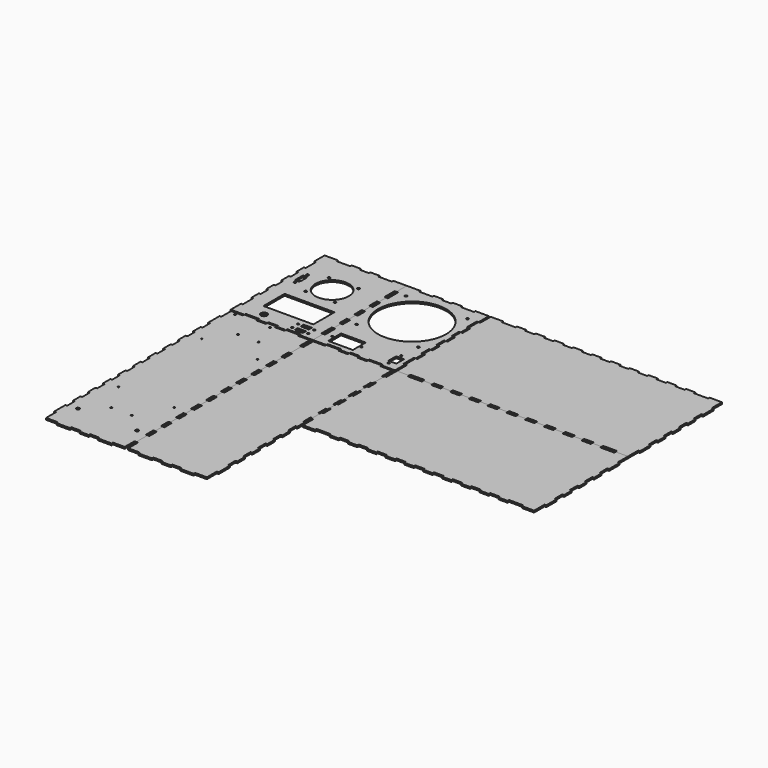
from build123d import *

# Parameters (mm, degrees)
F0_R     = 5.5001224188
F0_R_2   = 1.7501355185
F0_W     = 14
F0_H     = 6.5
F0_W_2   = 85
F0_H_2   = 45
F0_R_3   = 2.2023972195
F0_R_4   = 1.9999459509
F0_R_5   = 28.5
F1_DEPTH = 3
F0_R_6   = 2.75
F0_R_7   = 1.5
F0_R_8   = 1.25
F0_R_9   = 1.5001561361
F2_DEPTH = 3
F0_R_10  = 1.4999539677
F0_W_3   = 42
F0_H_3   = 27.5
F0_R_11  = 1.75
F0_W_4   = 13.5
F0_H_4   = 16.5
F0_R_12  = 1.9998336797
F0_R_13  = 58
F3_DEPTH = 3
F4_DEPTH = 3
F5_DEPTH = 3
F6_DEPTH = 3


# Not quite as in the source:
# - ends of sketch curves that miss each other by under 0.0002 mm in the source are joined


with BuildPart() as f1:
    # F0 (on Top) → F1 (new body)
    with BuildSketch(Plane.XY):
        Polygon((-317.001144, 300.00067), (-340.00059, 300.00067), (-340.00059, 278.00173), (-337.000596, 278.00173), (-337.000596, 256.00279), (-340.00059, 256.00279), (-340.00059, 240.00079), (-337.000596, 240.00079), (-337.000596, 223.99879), (-340.00059, 223.99879), (-340.00059, 207.99933), (-337.000596, 207.99933), (-337.000596, 191.99733), (-340.00059, 191.99733), (-340.00059, 175.99787), (-337.000596, 175.99787), (-337.000596, 159.99587), (-340.00059, 159.99587), (-340.00059, 144.00149), (-337.000596, 144.00149), (-337.000596, 122.00001), (-340.00059, 122.00001), (-340.00059, 100.00107), (-317.001144, 100.00107), (-317.001144, 102.99827), (-294.000174, 102.99827), (-294.000174, 100.00107), (-278.001222, 100.00107), (-278.001222, 102.99827), (-262.000746, 102.99827), (-262.000746, 100.00107), (-246.000524, 100.00107), (-246.000524, 102.99827), (-223.001078, 102.99827), (-223.001078, 100.00107), (-200.000108, 100.00107), (-200.000108, 122.00001), (-203.000102, 122.00001), (-203.000102, 144.00149), (-200.000108, 144.00149), (-200.000108, 159.99587), (-203.000102, 159.99587), (-203.000102, 175.99787), (-200.000108, 175.99787), (-200.000108, 191.99733), (-203.000102, 191.99733), (-203.000102, 207.99933), (-200.000108, 207.99933), (-200.000108, 223.99879), (-203.000102, 223.99879), (-203.000102, 240.00079), (-200.000108, 240.00079), (-200.000108, 256.00279), (-203.000102, 256.00279), (-203.000102, 278.00173), (-200.000108, 278.00173), (-200.000108, 300.00067), (-223.001078, 300.00067), (-223.001078, 297.00093), (-246.000524, 297.00093), (-246.000524, 300.00067), (-262.000746, 300.00067), (-262.000746, 297.00093), (-278.001222, 297.00093), (-278.001222, 300.00067), (-294.000174, 300.00067), (-294.000174, 297.00093), (-317.001144, 297.00093), align=None)
        with Locations((-296.856862573, 116.9972511531)):
            Circle(F0_R, mode=Mode.SUBTRACT)
        with Locations((-243.809402042, 110.6649048161)):
            Circle(F0_R_2, mode=Mode.SUBTRACT)
        with Locations((-230.059402042, 110.6915399432)):
            Rectangle(F0_W, F0_H, mode=Mode.SUBTRACT)
        with Locations((-216.309402042, 110.6649048161)):
            Circle(F0_R_2, mode=Mode.SUBTRACT)
        with Locations((-243.8093970094, 123.4562702011)):
            Circle(F0_R_2, mode=Mode.SUBTRACT)
        with Locations((-230.0593970094, 123.4829053283)):
            Rectangle(F0_W, F0_H, mode=Mode.SUBTRACT)
        with Locations((-216.3093970094, 123.4562702011)):
            Circle(F0_R_2, mode=Mode.SUBTRACT)
        with Locations((-270.001013279, 157.8700011969)):
            Rectangle(F0_W_2, F0_H_2, mode=Mode.SUBTRACT)
        with Locations((-322.4638801523, 215.0738120902)):
            Circle(F0_R_3, mode=Mode.SUBTRACT)
        with Locations((-295.0011516983, 203.4637744319)):
            Circle(F0_R_4, mode=Mode.SUBTRACT)
        with Locations((-245.0010429199, 203.4637744319)):
            Circle(F0_R_4, mode=Mode.SUBTRACT)
        Polygon((-318.3998801523, 222.5198170102), (-320.1778801523, 219.7258170102), (-326.5278801523, 219.7258170102), (-326.5278801523, 237.2258175702), (-320.1778801523, 237.2258175702), (-318.3998801523, 234.4318175702), align=None, mode=Mode.SUBTRACT)
        with Locations((-322.4638801523, 241.8778224902)):
            Circle(F0_R_3, mode=Mode.SUBTRACT)
        with Locations((-270.0010973091, 228.4637673539)):
            Circle(F0_R_5, mode=Mode.SUBTRACT)
        with Locations((-295.0011516983, 253.4637602758)):
            Circle(F0_R_4, mode=Mode.SUBTRACT)
        with Locations((-245.0010429199, 253.4637602758)):
            Circle(F0_R_4, mode=Mode.SUBTRACT)
    extrude(amount=F1_DEPTH)


with BuildPart() as f2:
    # F0 (on Top) → F2 (new body)
    with BuildSketch(Plane.XY):
        Polygon((-294.000174, 100.00107), (-317.001144, 100.00107), (-317.001144, 96.99879), (-337.000596, 96.99879), (-337.000596, 76.00061), (-340.00059, 76.00061), (-340.00059, 52.00015), (-337.000596, 52.00015), (-337.000596, 35.99815), (-340.00059, 35.99815), (-340.00059, 20.00123), (-337.000596, 20.00123), (-337.000596, 3.99923), (-340.00059, 3.99923), (-340.00059, -12.00023), (-337.000596, -12.00023), (-337.000596, -28.00223), (-340.00059, -28.00223), (-340.00059, -43.99915), (-337.000596, -43.99915), (-337.000596, -60.001404), (-340.00059, -60.001404), (-340.00059, -76.00061), (-337.000596, -76.00061), (-337.000596, -92.001086), (-340.00059, -92.001086), (-340.00059, -108.000038), (-337.000596, -108.000038), (-337.000596, -124.00153), (-340.00059, -124.00153), (-340.00059, -139.999466), (-337.000596, -139.999466), (-337.000596, -156.000958), (-340.00059, -156.000958), (-340.00059, -172.000164), (-337.000596, -172.000164), (-337.000596, -188.00191), (-340.00059, -188.00191), (-340.00059, -203.999592), (-337.000596, -203.999592), (-337.000596, -220.001338), (-340.00059, -220.001338), (-340.00059, -236.000544), (-337.000596, -236.000544), (-337.000596, -252.000766), (-340.00059, -252.000766), (-340.00059, -276.000718), (-337.0006056227, -276.000718), (-337.000596, -297.000676), (-317.001144, -297.000676), (-317.001144, -300.00067), (-294.000174, -300.00067), (-294.000174, -297.000676), (-278.001222, -297.000676), (-278.001222, -300.00067), (-262.000746, -300.00067), (-262.000746, -297.000676), (-246.000524, -297.000676), (-246.000524, -300.00067), (-223.001078, -300.00067), (-223.001078, -297.000676), (-203.000102, -297.000676), (-203.000102, -276.000718), (-200.000108, -276.000718), (-200.000108, -252.000766), (-203.000102, -252.000766), (-203.000102, -236.000544), (-200.000108, -236.000544), (-200.000108, -220.001338), (-203.000102, -220.001338), (-203.000102, -203.999592), (-200.000108, -203.999592), (-200.000108, -188.00191), (-203.000102, -188.00191), (-203.000102, -172.000164), (-200.000108, -172.000164), (-200.000108, -156.000958), (-203.000102, -156.000958), (-203.000102, -139.999466), (-200.000108, -139.999466), (-200.000108, -124.00153), (-203.000102, -124.00153), (-203.000102, -108.000038), (-200.000108, -108.000038), (-200.000108, -92.001086), (-203.000102, -92.001086), (-203.000102, -76.00061), (-200.000108, -76.00061), (-200.000108, -60.001404), (-203.000102, -60.001404), (-203.000102, -43.99915), (-200.000108, -43.99915), (-200.000108, -28.00223), (-203.000102, -28.00223), (-203.000102, -12.00023), (-200.000108, -12.00023), (-200.000108, 3.99923), (-203.000102, 3.99923), (-203.000102, 20.00123), (-200.000108, 20.00123), (-200.000108, 35.99815), (-203.000102, 35.99815), (-203.000102, 52.00015), (-200.000108, 52.00015), (-200.000108, 76.00061), (-203.000102, 76.00061), (-203.000102, 96.99879), (-223.001078, 96.99879), (-223.001078, 100.00107), (-246.000524, 100.00107), (-246.000524, 96.99879), (-262.000746, 96.99879), (-262.000746, 100.00107), (-278.001222, 100.00107), (-278.001222, 96.99879), (-294.000174, 96.99879), align=None)
        with Locations((-320.4981392353, -249.8400263762)):
            Circle(F0_R_6, mode=Mode.SUBTRACT)
        with Locations((-219.4981392353, -249.8400263762)):
            Circle(F0_R_6, mode=Mode.SUBTRACT)
        with Locations((-287.4827867562, -219.9880003408)):
            Circle(F0_R_7, mode=Mode.SUBTRACT)
        with Locations((-317.5006971111, -167.2832300663)):
            Circle(F0_R_8, mode=Mode.SUBTRACT)
        with Locations((-252.4827370386, -219.9884861494)):
            Circle(F0_R_7, mode=Mode.SUBTRACT)
        with Locations((-222.5006971111, -167.2832300663)):
            Circle(F0_R_8, mode=Mode.SUBTRACT)
        with Locations((-317.5006971111, 10.2167699337)):
            Circle(F0_R_8, mode=Mode.SUBTRACT)
        with Locations((-287.483402451, 50.0039782226)):
            Circle(F0_R_7, mode=Mode.SUBTRACT)
        with Locations((-222.5006971111, 10.2167699337)):
            Circle(F0_R_8, mode=Mode.SUBTRACT)
        with Locations((-252.4833581656, 50.0046229419)):
            Circle(F0_R_7, mode=Mode.SUBTRACT)
        with Locations((-326.6070187092, 92.3456028104)):
            Circle(F0_R_9, mode=Mode.SUBTRACT)
        with Locations((-267.1067064369, 92.3456028104)):
            Circle(F0_R_9, mode=Mode.SUBTRACT)
    extrude(amount=F2_DEPTH)


with BuildPart() as f3:
    # F0 (on Top) → F3 (new body)
    with BuildSketch(Plane.XY):
        Polygon((-177.000662, 300.00067), (-200.000108, 300.00067), (-200.000108, 278.00173), (-197.000368, 278.00173), (-197.000368, 256.00279), (-200.000108, 256.00279), (-200.000108, 240.00079), (-197.000368, 240.00079), (-197.000368, 223.99879), (-200.000108, 223.99879), (-200.000108, 207.99933), (-197.000368, 207.99933), (-197.000368, 191.99733), (-200.000108, 191.99733), (-200.000108, 175.99787), (-197.000368, 175.99787), (-197.000368, 159.99587), (-200.000108, 159.99587), (-200.000108, 144.00149), (-197.000368, 144.00149), (-197.000368, 122.00001), (-200.000108, 122.00001), (-200.000108, 100.00107), (-177.000662, 100.00107), (-177.000662, 102.99827), (-154.001216, 102.99827), (-154.001216, 100.00107), (-138.00074, 100.00107), (-138.00074, 102.99827), (-122.000518, 102.99827), (-122.000518, 100.00107), (-105.999788, 100.00107), (-105.999788, 102.99827), (-83.00085, 102.99827), (-83.00085, 100.00107), (-60.00115, 100.00107), (-60.00115, 122.00001), (-63.00089, 122.00001), (-63.00089, 144.00149), (-60.00115, 144.00149), (-60.00115, 159.99587), (-63.00089, 159.99587), (-63.00089, 175.99787), (-60.00115, 175.99787), (-60.00115, 191.99733), (-63.00089, 191.99733), (-63.00089, 207.99933), (-60.00115, 207.99933), (-60.00115, 223.99879), (-63.00089, 223.99879), (-63.00089, 240.00079), (-60.00115, 240.00079), (-60.00115, 256.00279), (-63.00089, 256.00279), (-63.00089, 278.00173), (-60.00115, 278.00173), (-60.00115, 300.00067), (-83.00085, 300.00067), (-83.00085, 297.00093), (-105.999788, 297.00093), (-105.999788, 300.00067), (-122.000518, 300.00067), (-122.000518, 297.00093), (-138.00074, 297.00093), (-138.00074, 300.00067), (-154.001216, 300.00067), (-154.001216, 297.00093), (-177.000662, 297.00093), align=None)
        with Locations((-186.41741882, 124.4014510885)):
            Circle(F0_R_10, mode=Mode.SUBTRACT)
        with Locations((-161.4174648523, 124.4014510885)):
            Rectangle(F0_W_3, F0_H_3, mode=Mode.SUBTRACT)
        with Locations((-136.4175108847, 124.4014510885)):
            Circle(F0_R_10, mode=Mode.SUBTRACT)
        with Locations((-79.6923562884, 110.8830720186)):
            Circle(F0_R_11, mode=Mode.SUBTRACT)
        with Locations((-77.4423562884, 124.3830720186)):
            Rectangle(F0_W_4, F0_H_4, mode=Mode.SUBTRACT)
        with Locations((-79.6923562884, 137.8830720186)):
            Circle(F0_R_11, mode=Mode.SUBTRACT)
        with Locations((-182.5013941237, 171.3342382262)):
            Circle(F0_R_12, mode=Mode.SUBTRACT)
        with Locations((-182.5013941237, 276.3342722009)):
            Circle(F0_R_12, mode=Mode.SUBTRACT)
        with Locations((-130.0012281247, 223.8342552135)):
            Circle(F0_R_13, mode=Mode.SUBTRACT)
        with Locations((-77.5010621258, 171.3342382262)):
            Circle(F0_R_12, mode=Mode.SUBTRACT)
        with Locations((-77.5010621258, 276.3342722009)):
            Circle(F0_R_12, mode=Mode.SUBTRACT)
    extrude(amount=F3_DEPTH)


with BuildPart() as f4:
    # F0 (on Top) → F4 (new body)
    with BuildSketch(Plane.XY):
        Polygon((-154.001216, 100.00107), (-177.000662, 100.00107), (-177.000662, 96.99879), (-197.000368, 96.99879), (-197.000368, 76.00061), (-200.000108, 76.00061), (-200.000108, 52.00015), (-197.000368, 52.00015), (-197.000368, 35.99815), (-200.000108, 35.99815), (-200.000108, 20.00123), (-197.000368, 20.00123), (-197.000368, 3.99923), (-200.000108, 3.99923), (-200.000108, -12.00023), (-197.000368, -12.00023), (-197.000368, -28.00223), (-200.000108, -28.00223), (-200.000108, -43.99915), (-197.000368, -43.99915), (-197.000368, -60.001404), (-200.000108, -60.001404), (-200.000108, -76.00061), (-197.000368, -76.00061), (-197.000368, -92.001086), (-200.000108, -92.001086), (-200.000108, -108.000038), (-197.000368, -108.000038), (-197.000368, -124.00153), (-200.000108, -124.00153), (-200.000108, -139.999466), (-197.000368, -139.999466), (-197.000368, -156.000958), (-200.000108, -156.000958), (-200.000108, -172.000164), (-197.000368, -172.000164), (-197.000368, -188.00191), (-200.000108, -188.00191), (-200.000108, -203.999592), (-197.000368, -203.999592), (-197.000368, -220.001338), (-200.000108, -220.001338), (-200.000108, -236.000544), (-197.000368, -236.000544), (-197.000368, -252.000766), (-200.000108, -252.000766), (-200.000108, -276.000718), (-197.000368, -276.000718), (-197.000368, -297.000676), (-177.000662, -297.000676), (-177.000662, -300.00067), (-154.001216, -300.00067), (-154.001216, -297.000676), (-138.00074, -297.000676), (-138.00074, -300.00067), (-122.000518, -300.00067), (-122.000518, -297.000676), (-105.999788, -297.000676), (-105.999788, -300.00067), (-83.00085, -300.00067), (-83.00085, -297.000676), (-63.00089, -297.000676), (-63.00089, -276.000718), (-60.00115, -276.000718), (-60.00115, -252.000766), (-63.00089, -252.000766), (-63.00089, -236.000544), (-60.00115, -236.000544), (-60.00115, -220.001338), (-63.00089, -220.001338), (-63.00089, -203.999592), (-60.00115, -203.999592), (-60.00115, -188.00191), (-63.00089, -188.00191), (-63.00089, -172.000164), (-60.00115, -172.000164), (-60.00115, -156.000958), (-63.00089, -156.000958), (-63.00089, -139.999466), (-60.00115, -139.999466), (-60.00115, -124.00153), (-63.00089, -124.00153), (-63.00089, -108.000038), (-60.00115, -108.000038), (-60.00115, -92.001086), (-63.00089, -92.001086), (-63.00089, -76.00061), (-60.00115, -76.00061), (-60.00115, -60.001404), (-63.00089, -60.001404), (-63.00089, -43.99915), (-60.00115, -43.99915), (-60.00115, -40.00119), (-60.00115, -28.00223), (-63.00089, -28.00223), (-63.00089, -12.00023), (-60.00115, -12.00023), (-60.00115, -7.99973), (-60.00115, 3.99923), (-63.00089, 3.99923), (-63.00089, 20.00123), (-60.00115, 20.00123), (-60.00115, 23.99919), (-60.00115, 35.99815), (-63.00089, 35.99815), (-63.00089, 52.00015), (-60.00115, 52.00015), (-60.00115, 56.00065), (-60.00115, 76.00061), (-63.00089, 76.00061), (-63.00089, 96.99879), (-83.00085, 96.99879), (-83.00085, 100.00107), (-105.999788, 100.00107), (-105.999788, 96.99879), (-122.000518, 96.99879), (-122.000518, 100.00107), (-138.00074, 100.00107), (-138.00074, 96.99879), (-154.001216, 96.99879), align=None)
    extrude(amount=F4_DEPTH)


with BuildPart() as f5:
    # F0 (on Top) → F5 (new body)
    with BuildSketch(Plane.XY):
        Polygon((-57.00141, 278.00173), (-60.00115, 278.00173), (-60.00115, 256.00279), (-57.00141, 256.00279), (-57.00141, 240.00079), (-60.00115, 240.00079), (-60.00115, 223.99879), (-57.00141, 223.99879), (-57.00141, 207.99933), (-60.00115, 207.99933), (-60.00115, 191.99733), (-57.00141, 191.99733), (-57.00141, 175.99787), (-60.00115, 175.99787), (-60.00115, 159.99587), (-57.00141, 159.99587), (-57.00141, 144.00149), (-60.00115, 144.00149), (-60.00115, 122.00001), (-57.00141, 122.00001), (-57.00141, 100.00107), (-36.00069, 100.00107), (-36.00069, 102.99827), (-12.00023, 102.99827), (-12.00023, 100.00107), (3.99923, 100.00107), (3.99923, 102.99827), (19.99869, 102.99827), (19.99869, 100.00107), (36.00069, 100.00107), (36.00069, 102.99827), (52.00015, 102.99827), (52.00015, 100.00107), (68.00215, 100.00107), (68.00215, 102.99827), (83.99907, 102.99827), (83.99907, 100.00107), (99.99853, 100.00107), (99.99853, 102.99827), (116.00053, 102.99827), (116.00053, 100.00107), (131.99745, 100.00107), (131.99745, 102.99827), (147.99945, 102.99827), (147.99945, 100.00107), (163.99891, 100.00107), (163.99891, 102.99827), (180.00091, 102.99827), (180.00091, 100.00107), (196.00037, 100.00107), (196.00037, 102.99827), (211.99729, 102.99827), (211.99729, 100.00107), (227.99929, 100.00107), (227.99929, 102.99827), (243.99875, 102.99827), (243.99875, 100.00107), (260.00075, 100.00107), (260.00075, 102.99827), (275.99767, 102.99827), (275.99767, 100.00107), (291.99967, 100.00107), (291.99967, 102.99827), (316.00013, 102.99827), (316.00013, 100.00107), (336.99831, 100.00107), (336.99831, 122.00001), (340.00059, 122.00001), (340.00059, 144.00149), (336.99831, 144.00149), (336.99831, 159.99587), (340.00059, 159.99587), (340.00059, 175.99787), (336.99831, 175.99787), (336.99831, 191.99733), (340.00059, 191.99733), (340.00059, 207.99933), (336.99831, 207.99933), (336.99831, 223.99879), (340.00059, 223.99879), (340.00059, 240.00079), (336.99831, 240.00079), (336.99831, 256.00279), (340.00059, 256.00279), (340.00059, 278.00173), (336.99831, 278.00173), (336.99831, 300.00067), (316.00013, 300.00067), (316.00013, 297.00093), (291.99967, 297.00093), (291.99967, 300.00067), (275.99767, 300.00067), (275.99767, 297.00093), (260.00075, 297.00093), (260.00075, 300.00067), (243.99875, 300.00067), (243.99875, 297.00093), (227.99929, 297.00093), (227.99929, 300.00067), (211.99729, 300.00067), (211.99729, 297.00093), (196.00037, 297.00093), (196.00037, 300.00067), (180.00091, 300.00067), (180.00091, 297.00093), (163.99891, 297.00093), (163.99891, 300.00067), (147.99945, 300.00067), (147.99945, 297.00093), (131.99745, 297.00093), (131.99745, 300.00067), (116.00053, 300.00067), (116.00053, 297.00093), (99.99853, 297.00093), (99.99853, 300.00067), (83.99907, 300.00067), (83.99907, 297.00093), (68.00215, 297.00093), (68.00215, 300.00067), (52.00015, 300.00067), (52.00015, 297.00093), (36.00069, 297.00093), (36.00069, 300.00067), (19.99869, 300.00067), (19.99869, 297.00093), (3.99923, 297.00093), (3.99923, 300.00067), (-12.00023, 300.00067), (-12.00023, 297.00093), (-36.00069, 297.00093), (-36.00069, 300.00067), (-57.00141, 300.00067), align=None)
    extrude(amount=F5_DEPTH)


with BuildPart() as f6:
    # F0 (on Top) → F6 (new body)
    with BuildSketch(Plane.XY):
        Polygon((-36.00069, 100.00107), (-57.00141, 100.00107), (-57.00141, 77.99959), (-60.00115, 77.99959), (-60.00115, 76.00061), (-60.00115, 56.00065), (-57.00141, 56.00065), (-57.00141, 39.99865), (-60.00115, 39.99865), (-60.00115, 35.99815), (-60.00115, 23.99919), (-57.00141, 23.99919), (-57.00141, 7.99973), (-60.00115, 7.99973), (-60.00115, 3.99923), (-60.00115, -7.99973), (-57.00141, -7.99973), (-57.00141, -23.99919), (-60.00115, -23.99919), (-60.00115, -28.00223), (-60.00115, -40.00119), (-57.00141, -40.00119), (-57.00141, -55.999888), (-60.00115, -55.999888), (-60.00115, -60.001404), (-60.00115, -76.00061), (-60.00115, -78.000098), (-57.00141, -78.000098), (-57.00141, -100.000308), (-36.00069, -100.000308), (-36.00069, -97.000314), (-12.00023, -97.000314), (-12.00023, -100.000308), (3.99923, -100.000308), (3.99923, -97.000314), (19.99869, -97.000314), (19.99869, -100.000308), (36.00069, -100.000308), (36.00069, -97.000314), (52.00015, -97.000314), (52.00015, -100.000308), (68.00215, -100.000308), (68.00215, -97.000314), (83.99907, -97.000314), (83.99907, -100.000308), (99.99853, -100.000308), (99.99853, -97.000314), (116.00053, -97.000314), (116.00053, -100.000308), (131.99745, -100.000308), (131.99745, -97.000314), (147.99945, -97.000314), (147.99945, -100.000308), (163.99891, -100.000308), (163.99891, -97.000314), (180.00091, -97.000314), (180.00091, -100.000308), (196.00037, -100.000308), (196.00037, -97.000314), (211.99729, -97.000314), (211.99729, -100.000308), (227.99929, -100.000308), (227.99929, -97.000314), (243.99875, -97.000314), (243.99875, -100.000308), (260.00075, -100.000308), (260.00075, -97.000314), (275.99767, -97.000314), (275.99767, -100.000308), (291.99967, -100.000308), (291.99967, -97.000314), (316.00013, -97.000314), (316.00013, -100.000308), (336.99831, -100.000308), (336.99831, -78.000098), (340.00059, -78.000098), (340.00059, -55.999888), (336.99831, -55.999888), (336.99831, -40.00119), (340.00059, -40.00119), (340.00059, -23.99919), (336.99831, -23.99919), (336.99831, -7.99973), (340.00059, -7.99973), (340.00059, 7.99973), (336.99831, 7.99973), (336.99831, 23.99919), (340.00059, 23.99919), (340.00059, 39.99865), (336.99831, 39.99865), (336.99831, 56.00065), (340.00059, 56.00065), (340.00059, 77.99959), (336.99831, 77.99959), (336.99831, 100.00107), (316.00013, 100.00107), (316.00013, 96.99879), (291.99967, 96.99879), (291.99967, 100.00107), (275.99767, 100.00107), (275.99767, 96.99879), (260.00075, 96.99879), (260.00075, 100.00107), (243.99875, 100.00107), (243.99875, 96.99879), (227.99929, 96.99879), (227.99929, 100.00107), (211.99729, 100.00107), (211.99729, 96.99879), (196.00037, 96.99879), (196.00037, 100.00107), (180.00091, 100.00107), (180.00091, 96.99879), (163.99891, 96.99879), (163.99891, 100.00107), (147.99945, 100.00107), (147.99945, 96.99879), (131.99745, 96.99879), (131.99745, 100.00107), (116.00053, 100.00107), (116.00053, 96.99879), (99.99853, 96.99879), (99.99853, 100.00107), (83.99907, 100.00107), (83.99907, 96.99879), (68.00215, 96.99879), (68.00215, 100.00107), (52.00015, 100.00107), (52.00015, 96.99879), (36.00069, 96.99879), (36.00069, 100.00107), (19.99869, 100.00107), (19.99869, 96.99879), (3.99923, 96.99879), (3.99923, 100.00107), (-12.00023, 100.00107), (-12.00023, 96.99879), (-36.00069, 96.99879), align=None)
    extrude(amount=F6_DEPTH)


solid = Compound([f1.part, f2.part, f3.part, f4.part, f5.part, f6.part])
